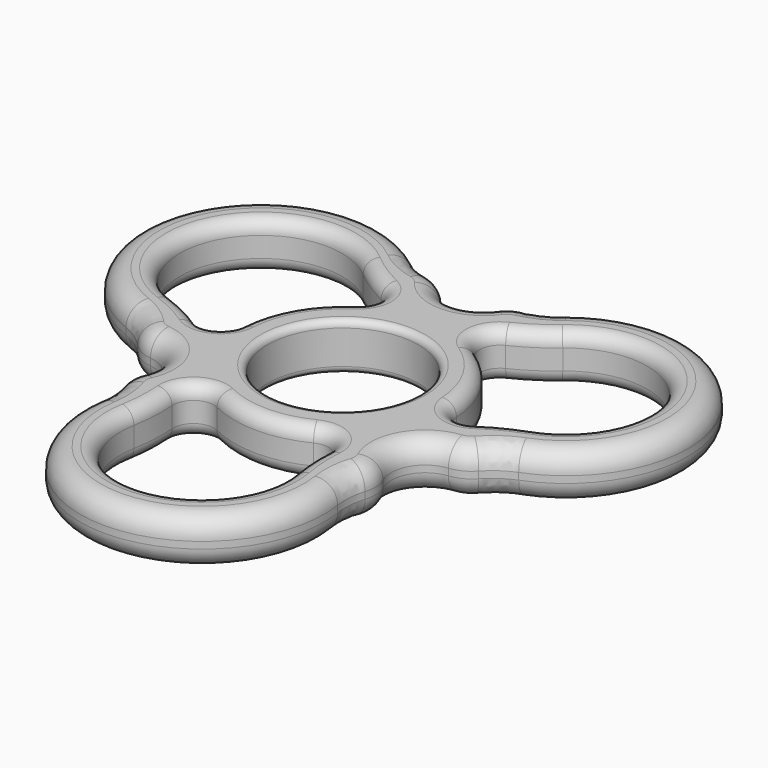
from build123d import *

# Parameters (mm, degrees)
F1_DEPTH  = 7
F2_R      = 18
F3_DEPTH  = 7
F4_R      = 11.15
F5_DEPTH  = 7.001
F7_DEPTH  = 7.001
F8_R      = 1
F9_R      = 10
F10_R     = 3
F12_DEPTH = 7.0010001
F13_R     = 2


with BuildPart() as f1:
    # F0 (on Top) → F1 (new body)
    with BuildSketch(Plane.XY):
        Polygon((0, 26), (-38.1051177665, 22), (38.1051177665, 22), align=None)
        Polygon((38.1051177665, 22), (-38.1051177665, 22), (0, -44), align=None)
        Polygon((0, -44), (-38.1051177665, 22), (-22.5166604984, -13), align=None)
        Polygon((22.5166604984, -13), (38.1051177665, 22), (0, -44), align=None)
    extrude(amount=F1_DEPTH)

    # F2 (on face) → F3 (join)
    with BuildSketch(Plane(origin=(0, 0, 0), x_dir=(1, 0, 0), z_dir=(0, 0, -1))):
        with Locations((-22.5166604984, -13)):
            Circle(F2_R)
        with Locations((22.5166604984, -13)):
            Circle(F2_R)
        with Locations((0, 26)):
            Circle(F2_R)
    extrude(amount=-F3_DEPTH)

    # F4 (on face) → F5 (cut, through all)
    with BuildSketch(Plane.XY.offset(7)):
        Circle(F4_R)
    extrude(amount=-F5_DEPTH, mode=Mode.SUBTRACT)

    # F6 (on face) → F7 (cut, through all)
    with BuildSketch(Plane.XY.offset(7)):
        with BuildLine():
            ThreePointArc((-8.612929891, 25.095876838), (-6.0566570255, 24.6906622679), (-4.04546707, 23.0615997234))
            ThreePointArc((-4.04546707, 23.0615997234), (0, 21), (4.04546707, 23.0615997234))
            ThreePointArc((4.04546707, 23.0615997234), (6.0566570255, 24.6906622679), (8.612929891, 25.095876838))
            Line((8.612929891, 25.095876838), (0, 26))
            Line((0, 26), (-8.612929891, 25.095876838))
        make_face()
        with BuildLine():
            Line((-22.5166604984, -13), (-17.4272019264, -20.0069545056))
            ThreePointArc((-17.4272019264, -20.0069545056), (-18.3544122475, -17.5905499801), (-17.9491976774, -15.0342771145))
            ThreePointArc((-17.9491976774, -15.0342771145), (-18.1865334795, -10.5), (-21.9946647474, -8.0273226089))
            ThreePointArc((-21.9946647474, -8.0273226089), (-24.411069273, -7.1001122878), (-26.0401318175, -5.0889223323))
            Line((-26.0401318175, -5.0889223323), (-22.5166604984, -13))
        make_face()
        with BuildLine():
            Line((22.5166604984, -13), (26.0401318175, -5.0889223323))
            ThreePointArc((26.0401318175, -5.0889223323), (24.411069273, -7.1001122878), (21.9946647474, -8.0273226089))
            ThreePointArc((21.9946647474, -8.0273226089), (18.1865334795, -10.5), (17.9491976774, -15.0342771145))
            ThreePointArc((17.9491976774, -15.0342771145), (18.3544122475, -17.5905499801), (17.4272019264, -20.0069545056))
            Line((17.4272019264, -20.0069545056), (22.5166604984, -13))
        make_face()
    extrude(amount=-F7_DEPTH, mode=Mode.SUBTRACT)

    # F8
    f8_edges = [f1.edges().sort_by_distance(p)[0] for p in [
        (-11.15, 0, 7),
        (11.15, 0, 3.5),
        (-11.15, 0, 0),
    ]]
    fillet(f8_edges, radius=F8_R)

    # F9
    f9_edges = [f1.edges().sort_by_distance(p)[0] for p in [
        (26.254492, -4.607629, 3.5),
        (17.949198, -15.034277, 3.5),
        (17.11757, -20.433243, 3.5),
        (-17.11757, -20.433243, 3.5),
        (-21.994665, -8.027323, 3.5),
        (-26.254492, -4.607629, 3.5),
        (-9.136922, 25.040872, 3.5),
        (-4.045467, 23.0616, 3.5),
        (9.136922, 25.040872, 3.5),
    ]]
    fillet(f9_edges, radius=F9_R)

    # F10
    f10_edges = [f1.edges().sort_by_distance(p)[0] for p in [
        (38.105118, 22, 0),
        (9.239804, 25.763401, 0),
        (26.931662, -4.879795, 0),
        (5.361077, 24.312218, 0),
        (23.735537, -7.513281, 0),
        (0, 21, 0),
        (18.186533, -10.5, 0),
        (-5.361077, 24.312218, 0),
        (18.37446, -16.798938, 0),
        (-9.239804, 25.763401, 0),
        (17.691858, -20.883606, 0),
        (-38.105118, 22, 0),
        (0, -44, 0),
        (-26.931662, -4.879795, 0),
        (-17.691858, -20.883606, 0),
        (-23.735537, -7.513281, 0),
        (-18.37446, -16.798938, 0),
        (-18.186533, -10.5, 0),
        (-12.15, 0, 0),
        (38.105118, 22, 7),
        (9.239804, 25.763401, 7),
        (26.931662, -4.879795, 7),
        (5.361077, 24.312218, 7),
        (23.735537, -7.513281, 7),
        (0, 21, 7),
        (18.186533, -10.5, 7),
        (-5.361077, 24.312218, 7),
        (18.37446, -16.798938, 7),
        (-9.239804, 25.763401, 7),
        (17.691858, -20.883606, 7),
        (-38.105118, 22, 7),
        (0, -44, 7),
        (-26.931662, -4.879795, 7),
        (-17.691858, -20.883606, 7),
        (-23.735537, -7.513281, 7),
        (-18.37446, -16.798938, 7),
        (-18.186533, -10.5, 7),
        (-12.15, 0, 7),
    ]]
    fillet(f10_edges, radius=F10_R)

    # F11 (on face) → F12 (cut, through all)
    with BuildSketch(Plane.XY.offset(7)):
        with BuildLine():
            ThreePointArc((7.121905551, -14.3275420545), (0, -16), (-7.121905551, -14.3275420545))
            ThreePointArc((-7.121905551, -14.3275420545), (-10.1305134502, -14.5239296032), (-11.4490844007, -17.235324117))
            ThreePointArc((-11.4490844007, -17.235324117), (-11.4156100675, -20.5480076413), (-11.8036435511, -23.8380566802))
            ThreePointArc((-11.8036435511, -23.8380566802), (0, -38), (11.8036435511, -23.8380566802))
            ThreePointArc((11.8036435511, -23.8380566802), (11.4156100675, -20.5480076413), (11.4490844007, -17.235324117))
            ThreePointArc((11.4490844007, -17.235324117), (10.1305134502, -14.5239296032), (7.121905551, -14.3275420545))
        make_face()
        with BuildLine():
            ThreePointArc((8.8470626175, 13.3315221577), (13.8564064606, 8), (15.9689681685, 0.9960198968))
            ThreePointArc((15.9689681685, 0.9960198968), (17.6433487243, -1.5113171997), (20.6507707282, -1.2975358826))
            ThreePointArc((20.6507707282, -1.2975358826), (23.5029016482, 0.3877955025), (26.5461844374, 1.6967731676))
            ThreePointArc((26.5461844374, 1.6967731676), (32.9089653438, 19), (14.7425408863, 22.1412835126))
            ThreePointArc((14.7425408863, 22.1412835126), (12.0872915808, 20.1602121387), (9.2016863274, 18.5328599996))
            ThreePointArc((9.2016863274, 18.5328599996), (7.5128352741, 16.0352468029), (8.8470626175, 13.3315221577))
        make_face()
        with BuildLine():
            ThreePointArc((-15.9689681685, 0.9960198968), (-13.8564064606, 8), (-8.8470626175, 13.3315221577))
            ThreePointArc((-8.8470626175, 13.3315221577), (-7.5128352741, 16.0352468029), (-9.2016863274, 18.5328599996))
            ThreePointArc((-9.2016863274, 18.5328599996), (-12.0872915808, 20.1602121387), (-14.7425408863, 22.1412835126))
            ThreePointArc((-14.7425408863, 22.1412835126), (-32.9089653438, 19), (-26.5461844374, 1.6967731676))
            ThreePointArc((-26.5461844374, 1.6967731676), (-23.5029016482, 0.3877955025), (-20.6507707282, -1.2975358826))
            ThreePointArc((-20.6507707282, -1.2975358826), (-17.6433487243, -1.5113171997), (-15.9689681685, 0.9960198968))
        make_face()
    extrude(amount=-F12_DEPTH, mode=Mode.SUBTRACT)

    # F13
    f13_edges = [f1.edges().sort_by_distance(p)[0] for p in [
        (35.507042, 20.5, 7),
        (10.533484, 23.056674, 7),
        (25.234407, -2.406072, 7),
        (6.998991, 21.798807, 7),
        (22.377816, -4.838099, 7),
        (0, 18, 7),
        (15.588457, -9, 7),
        (-6.998991, 21.798807, 7),
        (15.378825, -16.960708, 7),
        (-10.533484, 23.056674, 7),
        (14.700923, -20.650601, 7),
        (-35.507042, 20.5, 7),
        (0, -41, 7),
        (-25.234407, -2.406072, 7),
        (-14.700923, -20.650602, 7),
        (-22.377816, -4.838099, 7),
        (-15.378825, -16.960708, 7),
        (-15.588457, -9, 7),
        (-23.502902, 0.387796, 7),
        (-32.908965, 19, 7),
        (-12.087292, 20.160212, 7),
        (-7.512835, 16.035247, 7),
        (-13.856406, 8, 7),
        (-17.643349, -1.511317, 7),
        (-12.15, 0, 7),
        (12.087292, 20.160212, 7),
        (32.908965, 19, 7),
        (23.502902, 0.387796, 7),
        (17.643349, -1.511317, 7),
        (13.856406, 8, 7),
        (7.512835, 16.035247, 7),
        (11.41561, -20.548008, 7),
        (0, -38, 7),
        (-11.41561, -20.548008, 7),
        (-10.130513, -14.52393, 7),
        (0, -16, 7),
        (10.130513, -14.52393, 7),
        (35.507042, 20.5, 0),
        (10.533484, 23.056674, 0),
        (25.234407, -2.406072, 0),
        (6.998991, 21.798807, 0),
        (22.377816, -4.838099, 0),
        (0, 18, 0),
        (15.588457, -9, 0),
        (-6.998991, 21.798807, 0),
        (15.378825, -16.960708, 0),
        (-10.533484, 23.056674, 0),
        (14.700923, -20.650601, 0),
        (-35.507042, 20.5, 0),
        (0, -41, 0),
        (-25.234407, -2.406072, 0),
        (-14.700923, -20.650602, 0),
        (-22.377816, -4.838099, 0),
        (-15.378825, -16.960708, 0),
        (-15.588457, -9, 0),
        (10.130513, -14.52393, 0),
        (0, -16, 0),
        (-10.130513, -14.52393, 0),
        (-11.41561, -20.548008, 0),
        (0, -38, 0),
        (11.41561, -20.548008, 0),
        (-12.15, 0, 0),
        (-17.643349, -1.511317, 0),
        (-13.856406, 8, 0),
        (-7.512835, 16.035247, 0),
        (-12.087292, 20.160212, 0),
        (-32.908965, 19, 0),
        (-23.502902, 0.387796, 0),
        (7.512835, 16.035247, 0),
        (13.856406, 8, 0),
        (17.643349, -1.511317, 0),
        (23.502902, 0.387796, 0),
        (32.908965, 19, 0),
        (12.087292, 20.160212, 0),
    ]]
    fillet(f13_edges, radius=F13_R)


solid = f1.part
